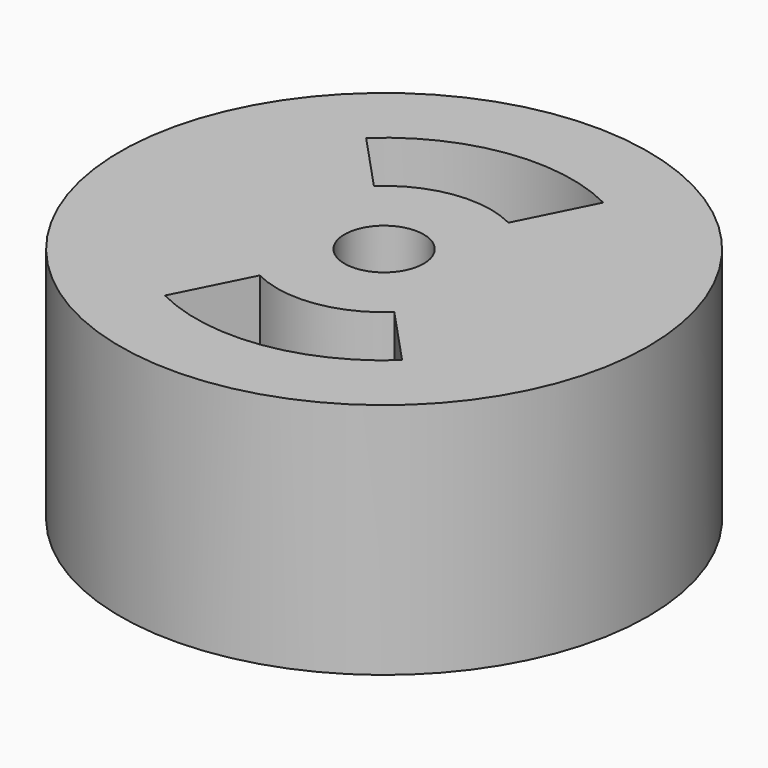
from build123d import *

# Parameters (mm, degrees)
F0_R     = 10
F0_R_2   = 1.5
F1_DEPTH = 9


# Not quite as in the source:
# - a feature names something its author has since deleted; it is built from what else it names


with BuildPart() as f1:
    # F0 (on Top) → F1 (new body)
    with BuildSketch(Plane.XY):
        Circle(F0_R)
        with BuildLine():
            Line((-3.2035890311, -6.37527581), (-1.8173406245, -3.6165836534))
            ThreePointArc((-1.8173406245, -3.6165836534), (0.5722008428, -4.0068679119), (2.756987683, -2.9633466189))
            Line((2.756987683, -2.9633466189), (4.8599890306, -5.2237564028))
            ThreePointArc((4.8599890306, -5.2237564028), (1.0086696565, -7.0632648157), (-3.2035890311, -6.37527581))
        make_face(mode=Mode.SUBTRACT)
        with BuildLine():
            ThreePointArc((-4.8599890306, 5.2237564028), (-1.0086696565, 7.0632648157), (3.2035890311, 6.37527581))
            Line((3.2035890311, 6.37527581), (1.8173406245, 3.6165836534))
            ThreePointArc((1.8173406245, 3.6165836534), (-0.5722008428, 4.0068679119), (-2.756987683, 2.9633466189))
            Line((-2.756987683, 2.9633466189), (-4.8599890306, 5.2237564028))
        make_face(mode=Mode.SUBTRACT)
        Circle(F0_R_2, mode=Mode.SUBTRACT)
    extrude(amount=F1_DEPTH)


solid = f1.part
